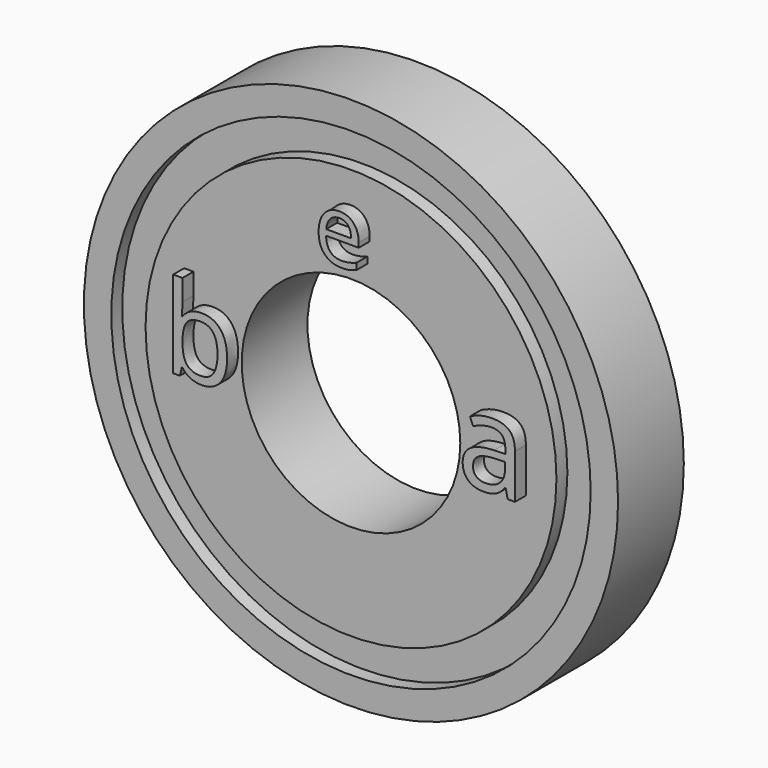
from build123d import *

# Parameters (mm, degrees)
F0_R           = 19.5
F1_DEPTH       = 2.5
F2_R           = 19.5
F2_R_2         = 17.5
F2_R_3         = 15
F3_DEPTH       = 1
F5_R           = 7.9797425055
F6_DEPTH       = 6.001
F7_TEXT_SIZE   = 8.3512932179
F7_TEXT_SIZE_2 = 6.4655181227
F7_TEXT_SIZE_3 = 8.8902201646
F8_DEPTH       = 1


# Not quite as in the source:
# - Text() gives the source's letters only with a copy of the font that has no kerning and outlines rounded to 1/6400 em; it was checked with that copy


with BuildPart() as f1:
    # F0 (on Front) → F1 (new body, symmetric)
    with BuildSketch(Plane.XZ):
        Circle(F0_R)
    extrude(amount=F1_DEPTH, both=True)

    # F2 (on face) → F3 (join)
    with BuildSketch(Plane.XZ.offset(2.5)):
        Circle(F2_R)
        Circle(F2_R_2, mode=Mode.SUBTRACT)
        Circle(F2_R_3)
    extrude(amount=F3_DEPTH)

    # F5 (on face) → F6 (cut, through all)
    with BuildSketch(Plane.XZ.offset(3.5)):
        Circle(F5_R)
    extrude(amount=-F6_DEPTH, mode=Mode.SUBTRACT)

    # F7 (on face) → F8 (join)
    with BuildSketch(Plane.XZ.offset(3.5)):
        with Locations((-12.8987077624, -1.6487069661)):
            Text('b', F7_TEXT_SIZE, font='Open Sans', text_align=(TextAlign.LEFT, TextAlign.BOTTOM))
        with Locations((-1.9265399314, 9.1871628538)):
            Text('e', F7_TEXT_SIZE_2, font='Open Sans', text_align=(TextAlign.LEFT, TextAlign.BOTTOM))
        with Locations((8.5471225902, -1.80096447)):
            Text('a', F7_TEXT_SIZE_3, font='Open Sans', text_align=(TextAlign.LEFT, TextAlign.BOTTOM))
    extrude(amount=F8_DEPTH)


solid = f1.part
